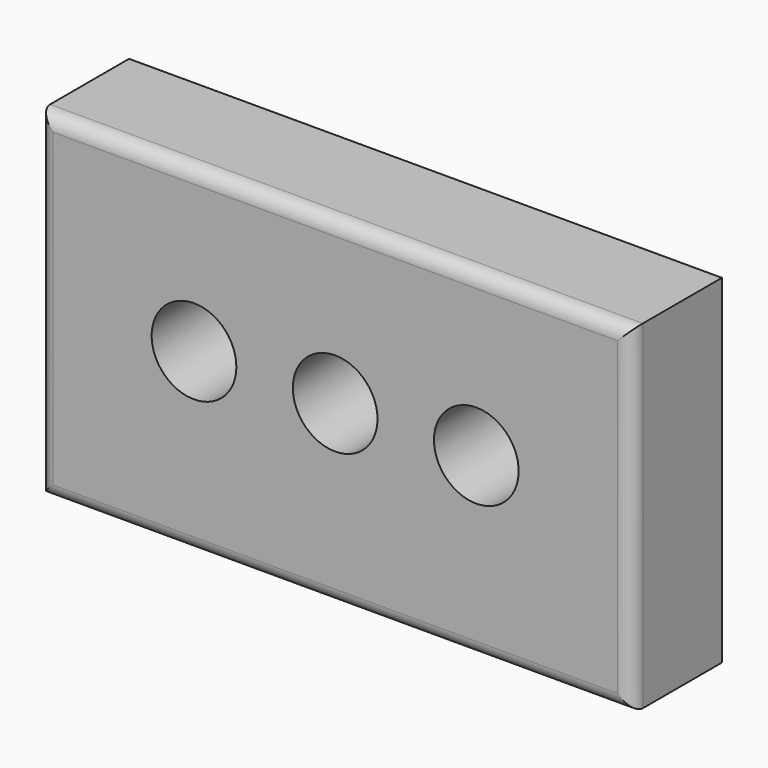
from build123d import *

# Parameters (mm, degrees)
F0_W     = 266.7
F0_H     = 152.4
F0_R     = 19.05
F1_DEPTH = 50.8
F2_DEPTH = 12.7
F3_R     = 6.35


with BuildPart() as f1:
    # F0 (on Front) → F1 (new body)
    with BuildSketch(Plane.XZ):
        Rectangle(F0_W, F0_H)
        with Locations((-63.5, 3.7267601583)):
            Circle(F0_R, mode=Mode.SUBTRACT)
        with BuildLine():
            ThreePointArc((-19.05, 3.7267601583), (0, 22.7767601583), (19.05, 3.7267601583))
            ThreePointArc((19.05, 3.7267601583), (0, -15.3232398417), (-19.05, 3.7267601583))
        make_face(mode=Mode.SUBTRACT)
        with BuildLine():
            ThreePointArc((82.55, 3.7267601583), (63.5, -15.3232398417), (44.45, 3.7267601583))
            ThreePointArc((44.45, 3.7267601583), (63.5, 22.7767601583), (82.55, 3.7267601583))
        make_face(mode=Mode.SUBTRACT)
    extrude(amount=F1_DEPTH)

    # F0 (on Front) → F2 (join)
    with BuildSketch(Plane.XZ):
        with BuildLine():
            ThreePointArc((-19.05, 3.7267601583), (0, -15.3232398417), (19.05, 3.7267601583))
            ThreePointArc((19.05, 3.7267601583), (0, 22.7767601583), (-19.05, 3.7267601583))
        make_face()
        with Locations((-63.5, 3.7267601583)):
            Circle(F0_R)
        with BuildLine():
            ThreePointArc((82.55, 3.7267601583), (63.5, 22.7767601583), (44.45, 3.7267601583))
            ThreePointArc((44.45, 3.7267601583), (63.5, -15.3232398417), (82.55, 3.7267601583))
        make_face()
    extrude(amount=F2_DEPTH)

    # F3
    f3_edges = [f1.edges().sort_by_distance(p)[0] for p in [
        (-133.35, -50.8, 0),
        (0, -50.8, -76.2),
        (133.35, -50.8, 0),
        (0, -50.8, 76.2),
    ]]
    fillet(f3_edges, radius=F3_R)


solid = f1.part
